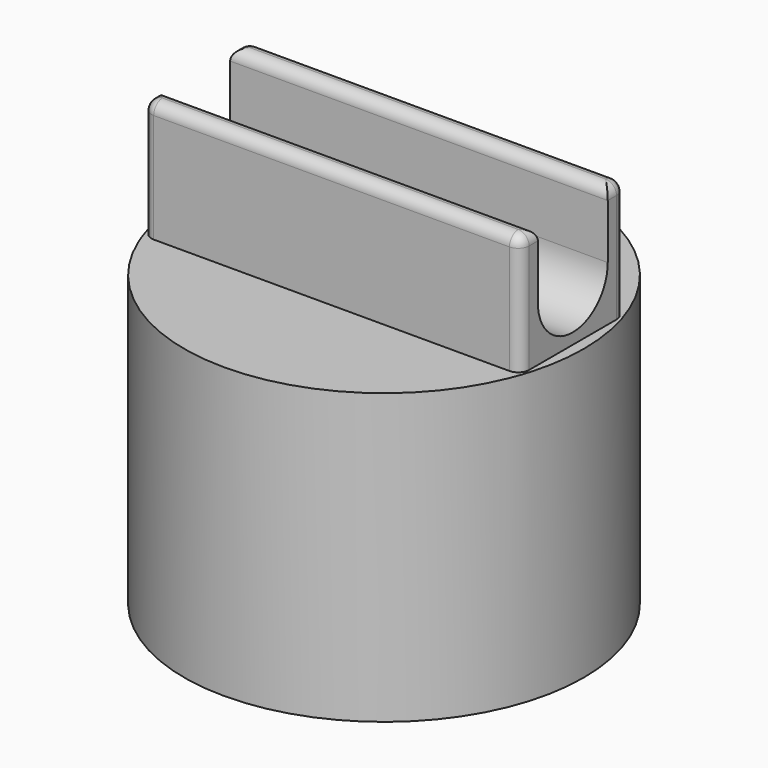
from build123d import *

# Parameters (mm, degrees)
F0_R         = 18.3
F0_R_2       = 16.8
F1_DEPTH     = 25
F2_R         = 18.3
F2_R_2       = 16.8
F3_DEPTH     = 1.5
F4_W         = 34.5768708821
F4_H         = 12
F5_DEPTH     = 5
F7_DEPTH     = 36
F8_W         = 34.5768708821
F8_H         = 2
F7_FACE_W    = 34.5768708821
F7_FACE_H    = 2
F9_DEPTH     = 6
F10_R        = 0.99999
F11_T1_DEPTH = 11
F11_T4_ANGLE = 90
F12_R        = 0.5


# Not quite as in the source:
# - a fillet or chamfer that OpenCascade refuses, or shapes differently, is made with other operations: its cross-section is extruded or revolved along the edge and cut away or added
# - a fillet or chamfer is up to 0.001 mm smaller than in the source, because OpenCascade refuses the exact size


with BuildPart() as f1:
    # F0 (on Top) → F1 (new body)
    with BuildSketch(Plane.XY):
        Circle(F0_R)
        Circle(F0_R_2, mode=Mode.SUBTRACT)
    extrude(amount=F1_DEPTH)

    # F2 (on face) → F3 (join)
    with BuildSketch(Plane.XY.offset(25)):
        Circle(F2_R)
        Circle(F2_R_2, mode=Mode.SUBTRACT)
        Circle(F2_R_2)
    extrude(amount=F3_DEPTH)

    # F4 (on face) → F5 (join)
    with BuildSketch(Plane.XY.offset(26.5)):
        Rectangle(F4_W, F4_H)
    extrude(amount=F5_DEPTH)

    # F6 (on face) → F7 (cut)
    with BuildSketch(Plane.YZ.offset(17.2884354411)):
        with BuildLine():
            ThreePointArc((-4, 31.5), (0, 27.5), (4, 31.5))
            Line((4, 31.5), (-4, 31.5))
        make_face()
    extrude(amount=-F7_DEPTH, mode=Mode.SUBTRACT)

    # F8 (on face) + F7_face (on face) → F9 (join)
    with BuildSketch(Plane.XY.offset(31.5)):
        with Locations((0, -5)):
            Rectangle(F8_W, F8_H)
    with BuildSketch(Plane(origin=(0, -5, 31.5), x_dir=(1, 0, 0), z_dir=(0, 0, 1))):
        with Locations((0, 10)):
            Rectangle(F7_FACE_W, F7_FACE_H)
    extrude(amount=F9_DEPTH)

    # F10 (radius 1 in the source; OpenCascade refuses exactly that, so slightly less here)
    f10_edges = [f1.edges().sort_by_distance(p)[0] for p in [
        (17.288435, -5, 37.5),
        (0, -4, 37.5),
        (-17.288435, -5, 37.5),
        (0, -6, 37.5),
        (-17.288435, 5, 37.5),
        (0, 4, 37.5),
        (17.288435, 5, 37.5),
        (0, 6, 37.5),
        (17.288435, -6, 32),
        (-17.288435, -6, 32),
        (-17.288435, 6, 32),
    ]]
    fillet(f10_edges, radius=F10_R)

    # F11: fillet of radius 1 on 1 edges, made by hand

    # F11_s2 → F11_t1 (cut)
    with BuildSketch(Plane.XY.offset(26.5)):
        with BuildLine():
            ThreePointArc((17.2884354411, 5), (16.9955422223, 5.7071067812), (16.2884354411, 6))
            Line((16.2884354411, 6), (17.2884354411, 6))
            Line((17.2884354411, 6), (17.2884354411, 5))
        make_face()
    extrude(amount=F11_T1_DEPTH, mode=Mode.SUBTRACT)

    # F11_s3 → F11_t4 (revolve, cut)
    with BuildSketch(Plane.XZ.offset(-5)):
        with BuildLine():
            ThreePointArc((16.2884454411, 37.5), (16.9955451512, 37.2071097101), (17.2884354411, 36.50001))
            Line((17.2884354411, 36.50001), (17.2884354411, 37.5))
            Line((17.2884354411, 37.5), (16.2884454411, 37.5))
        make_face()
    revolve(axis=Axis((16.2884354411, 5, 37.5), (0, 0, 1)), revolution_arc=F11_T4_ANGLE, mode=Mode.SUBTRACT)

    # F12
    f12_edges = [f1.edges().sort_by_distance(p)[0] for p in [
        (-16.8, 0, 0),
    ]]
    fillet(f12_edges, radius=F12_R)


solid = f1.part
